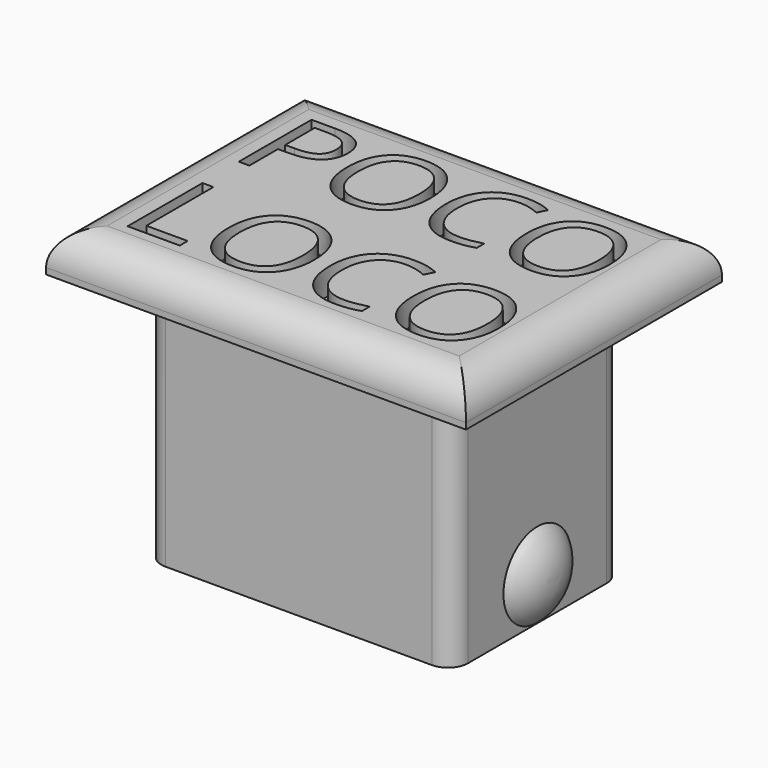
from build123d import *

# Parameters (mm, degrees)
F0_W           = 63
F0_H           = 48
F1_DEPTH       = 6
F3_DEPTH       = 38.1
F4_R           = 5.08
F5_TEXT_SIZE   = 19.0883471259
F5_TEXT_SIZE_2 = 19.672448568
F6_DEPTH       = 3.81
F7_DEPTH       = 25.4


# Not quite as in the source:
# - Text() gives the source's letters only with a copy of the font that has no kerning and outlines rounded to 1/6400 em; it was checked with that copy


with BuildPart() as f1:
    # F0 (on Top) → F1 (new body)
    with BuildSketch(Plane.XY):
        Rectangle(F0_W, F0_H)
    extrude(amount=F1_DEPTH)

    # F2 (on face) → F3 (join)
    with BuildSketch(Plane(origin=(0, 0, 0), x_dir=(1, 0, 0), z_dir=(0, 0, -1))):
        with BuildLine():
            Line((-20, -16), (20, -16))
            ThreePointArc((20, -16), (22.1213203436, -15.1213203436), (23, -13))
            Line((23, -13), (23, -6.1394460499))
            Line((23, -6.1394460499), (23, -4.9237548374))
            Line((23, -4.9237548374), (23, 4.2720362544))
            Line((23, 4.2720362544), (23, 5.3168511949))
            Line((23, 5.3168511949), (23, 13))
            ThreePointArc((23, 13), (22.1213203436, 15.1213203436), (20, 16))
            Line((20, 16), (-20, 16))
            ThreePointArc((-20, 16), (-22.1213203436, 15.1213203436), (-23, 13))
            Line((-23, 13), (-23, 5.4118060507))
            Line((-23, 5.4118060507), (-23, 4.4618933462))
            Line((-23, 4.4618933462), (-23, -4.1664787568))
            Line((-23, -4.1664787568), (-23, -5.2747102454))
            Line((-23, -5.2747102454), (-23, -13))
            ThreePointArc((-23, -13), (-22.1213203436, -15.1213203436), (-20, -16))
        make_face()
        Polygon((20, -6.1394460499), (20, -13), (-20, -13), (-20, -5.2747102454), (-20, -4.1664787568), (-20, 4.4618933462), (-20, 5.4118060507), (-20, 13), (20, 13), (20, 5.3168511949), (20, 4.2720362544), (20, -4.9237548374), align=None, mode=Mode.SUBTRACT)
    extrude(amount=F3_DEPTH)

    # F4
    f4_edges = [f1.edges().sort_by_distance(p)[0] for p in [
        (-31.5, 0, 6),
        (0, 24, 6),
        (31.5, 0, 6),
        (0, -24, 6),
    ]]
    fillet(f4_edges, radius=F4_R)

    # F5 (on face) → F6 (cut)
    with BuildSketch(Plane.XY.offset(6)):
        with Locations((-26.42, 3.456634864)):
            Text('POCO', F5_TEXT_SIZE, font='Open Sans', text_align=(TextAlign.LEFT, TextAlign.BOTTOM))
        with Locations((-26.42, -17.4771657552)):
            Text('LOCO', F5_TEXT_SIZE_2, font='Open Sans', text_align=(TextAlign.LEFT, TextAlign.BOTTOM))
    extrude(amount=-F6_DEPTH, mode=Mode.SUBTRACT)

    # F2 (on face) → F7 (join)
    with BuildSketch(Plane(origin=(0, 0, 0), x_dir=(1, 0, 0), z_dir=(0, 0, -1))):
        with BuildLine():
            Line((-20, -16), (20, -16))
            ThreePointArc((20, -16), (22.1213203436, -15.1213203436), (23, -13))
            Line((23, -13), (23, -6.1394460499))
            Line((23, -6.1394460499), (23, -4.9237548374))
            Line((23, -4.9237548374), (23, 4.2720362544))
            Line((23, 4.2720362544), (23, 5.3168511949))
            Line((23, 5.3168511949), (23, 13))
            ThreePointArc((23, 13), (22.1213203436, 15.1213203436), (20, 16))
            Line((20, 16), (-20, 16))
            ThreePointArc((-20, 16), (-22.1213203436, 15.1213203436), (-23, 13))
            Line((-23, 13), (-23, 5.4118060507))
            Line((-23, 5.4118060507), (-23, 4.4618933462))
            Line((-23, 4.4618933462), (-23, -4.1664787568))
            Line((-23, -4.1664787568), (-23, -5.2747102454))
            Line((-23, -5.2747102454), (-23, -13))
            ThreePointArc((-23, -13), (-22.1213203436, -15.1213203436), (-20, -16))
        make_face()
        Polygon((20, -6.1394460499), (20, -13), (-20, -13), (-20, -5.2747102454), (-20, -4.1664787568), (-20, 4.4618933462), (-20, 5.4118060507), (-20, 13), (20, 13), (20, 5.3168511949), (20, 4.2720362544), (20, -4.9237548374), align=None, mode=Mode.SUBTRACT)
    extrude(amount=F7_DEPTH)

    # F8 (on Front) → F9 (revolve)
    with BuildSketch(Plane.XZ):
        with BuildLine():
            ThreePointArc((-25.3194807459, -31.6491123611), (-24.7693085128, -34.7662414657), (-23, -37.390880627))
            Line((-23, -37.390880627), (-23, -31.6491123611))
            Line((-23, -31.6491123611), (-25.3194807459, -31.6491123611))
        make_face()
    revolve(axis=Axis((-24.159740373, 0, -31.6491123611), (-1, 0, 0)))

    # F10 (on Front) → F11 (revolve)
    with BuildSketch(Plane.XZ):
        with BuildLine():
            Line((23, -31.6681114107), (23, -38.0181114107))
            ThreePointArc((23, -38.0181114107), (25.1415853152, -35.1743596212), (25.7576497511, -31.6681114107))
            Line((25.7576497511, -31.6681114107), (23, -31.6681114107))
        make_face()
    revolve(axis=Axis((24.3788248755, 0, -31.6681114107), (1, 0, 0)))


solid = f1.part
